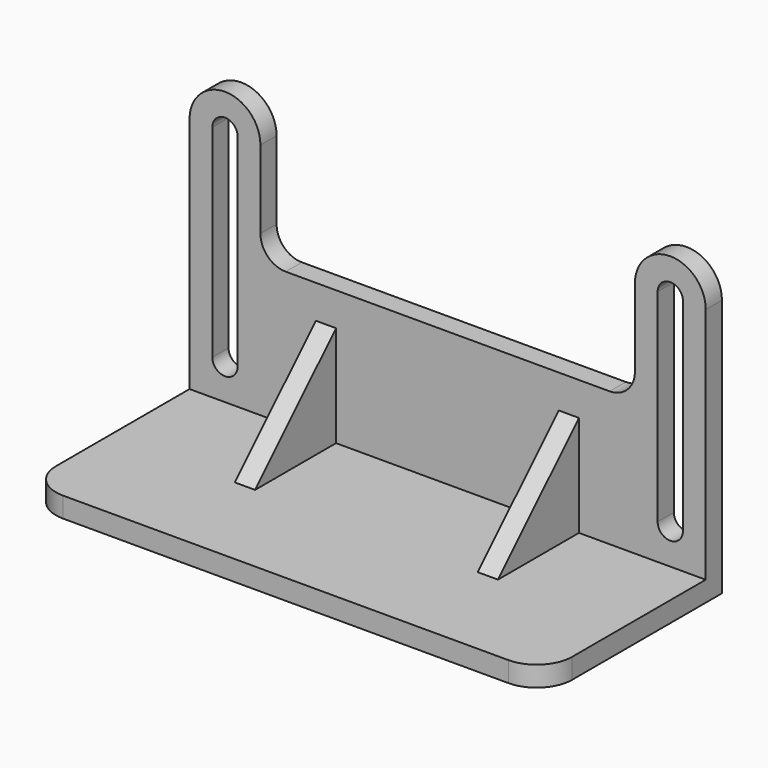
from build123d import *

# Parameters (mm, degrees)
F1_DEPTH = 5.08
F0_W     = 129.5400008702
F0_H     = 5.08
F2_DEPTH = 55.88
F4_DEPTH = 5.08
F6_START = 30.48
F6_DEPTH = 5.08
F7_START = -25.4
F7_DEPTH = 5.08


# Not quite as in the source:
# - a feature names something its author has since deleted; it is built from what else it names


with BuildPart() as f1:
    # F0 (on Front) → F1 (new body)
    with BuildSketch(Plane.XZ):
        with BuildLine():
            Line((-62.1654726565, 25.9080137503), (-62.1654726565, -33.7819862497))
            Line((-62.1654726565, -33.7819862497), (67.3745282138, -33.7819862497))
            Line((67.3745282138, -33.7819862497), (67.3745282138, 25.9080137503))
            ThreePointArc((67.3745282138, 25.9080137503), (58.4845213386, 34.7980137503), (49.5945282137, 25.908))
            Line((49.5945282137, 25.908), (49.5945282137, 6.35))
            ThreePointArc((49.5945282137, 6.35), (47.7346562743, 1.8598719395), (43.2445282137, 0))
            Line((43.2445282137, 0), (-38.0354726565, 0))
            ThreePointArc((-38.0354726565, 0), (-42.525600717, 1.8598719395), (-44.3854726565, 6.35))
            Line((-44.3854726565, 6.35), (-44.3854726565, 25.908))
            ThreePointArc((-44.3854726565, 25.908), (-53.2754657813, 34.7980137503), (-62.1654726565, 25.9080137503))
        make_face()
        with BuildLine():
            ThreePointArc((-56.4504726565, 25.9080137503), (-53.2754726565, 29.0830137503), (-50.1004726565, 25.9080137503))
            Line((-50.1004726565, 25.9080137503), (-50.1004726565, -24.8919862497))
            ThreePointArc((-50.1004726565, -24.8919862497), (-53.2754726565, -28.0669862497), (-56.4504726565, -24.8919862497))
            Line((-56.4504726565, -24.8919862497), (-56.4504726565, 25.9080137503))
        make_face(mode=Mode.SUBTRACT)
        with BuildLine():
            ThreePointArc((55.3095273435, 25.9080137503), (58.4845273435, 29.0830137503), (61.6595273435, 25.9080137503))
            Line((61.6595273435, 25.9080137503), (61.6595273435, -24.8919862497))
            ThreePointArc((61.6595273435, -24.8919862497), (58.4845273435, -28.0669862497), (55.3095273435, -24.8919862497))
            Line((55.3095273435, -24.8919862497), (55.3095273435, 25.9080137503))
        make_face(mode=Mode.SUBTRACT)
    extrude(amount=F1_DEPTH)

    # F0 (on Front) → F2 (join)
    with BuildSketch(Plane.XZ):
        with Locations((2.6045277786, -36.3219862497)):
            Rectangle(F0_W, F0_H)
    extrude(amount=F2_DEPTH)

    # F3 (on face) → F4 (cut)
    with BuildSketch(Plane.XY.offset(-33.7819862497)):
        with BuildLine():
            ThreePointArc((-53.2754726565, -55.88), (-59.5616519412, -53.2761792847), (-62.1654726565, -46.99))
            Line((-62.1654726565, -46.99), (-62.1654726565, -55.88))
            Line((-62.1654726565, -55.88), (-53.2754726565, -55.88))
        make_face()
        with BuildLine():
            ThreePointArc((67.3745282138, -46.99), (64.7707071908, -53.2761795924), (58.4845273435, -55.88))
            Line((58.4845273435, -55.88), (67.3745282138, -55.88))
            Line((67.3745282138, -55.88), (67.3745282138, -46.99))
        make_face()
    extrude(amount=-F4_DEPTH, mode=Mode.SUBTRACT)

    # F5 (on Right) → F6 (join)
    with BuildSketch(Plane.YZ.offset(F6_START)):
        Polygon((-5.08, -33.7819862497), (-5.08, -8.3819862497), (-30.48, -33.7819862497), align=None)
    extrude(amount=F6_DEPTH)

    # F5 (on Right) → F7 (join)
    with BuildSketch(Plane.YZ.offset(F7_START)):
        Polygon((-5.08, -33.7819862497), (-5.08, -8.3819862497), (-30.48, -33.7819862497), align=None)
    extrude(amount=-F7_DEPTH)


solid = f1.part
